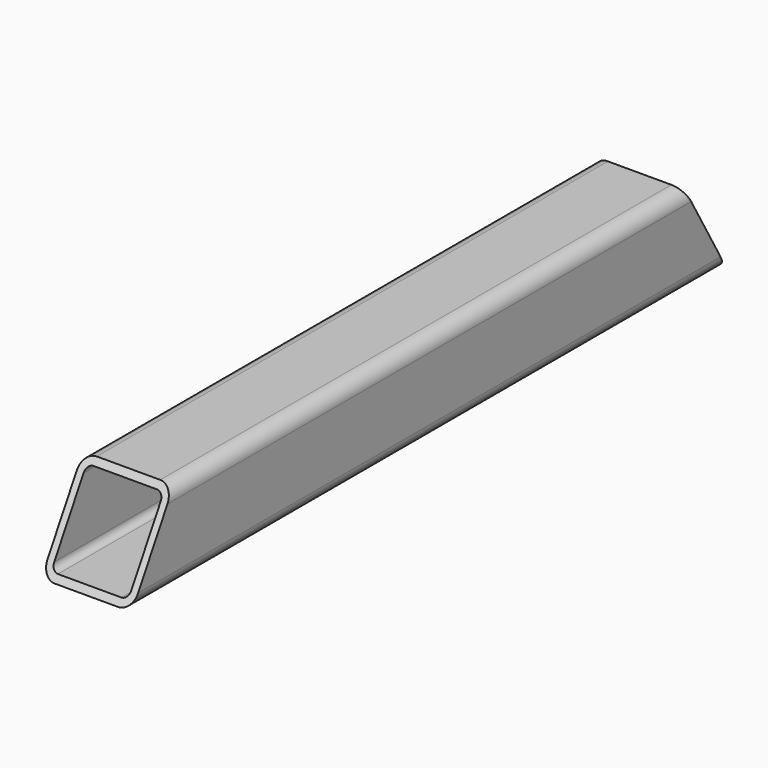
from build123d import *

# Parameters (mm, degrees)
F1_DEPTH = 1041.4
F3_DEPTH = 127.001


# Not quite as in the source:
# - a feature names something its author has since deleted; it is built from what else it names


with BuildPart() as f1:
    # F0 (on Front) → F1 (new body)
    with BuildSketch(Plane.XZ):
        with BuildLine():
            ThreePointArc((0, 19.05), (5.5796158184, 5.5796158184), (19.05, 0))
            Line((19.05, 0), (107.95, 0))
            ThreePointArc((107.95, 0), (121.4203841816, 5.5796158184), (127, 19.05))
            Line((127, 19.05), (127, 107.95))
            ThreePointArc((127, 107.95), (121.4203841816, 121.4203841816), (107.95, 127))
            Line((107.95, 127), (19.05, 127))
            ThreePointArc((19.05, 127), (5.5796158184, 121.4203841816), (0, 107.95))
            Line((0, 107.95), (0, 19.05))
        make_face()
        with BuildLine():
            ThreePointArc((19.05, 9.525), (12.3148079092, 12.3148079092), (9.525, 19.05))
            Line((9.525, 19.05), (9.525, 107.95))
            ThreePointArc((9.525, 107.95), (12.3148079092, 114.6851920908), (19.05, 117.475))
            Line((19.05, 117.475), (107.95, 117.475))
            ThreePointArc((107.95, 117.475), (114.6851920908, 114.6851920908), (117.475, 107.95))
            Line((117.475, 107.95), (117.475, 19.05))
            ThreePointArc((117.475, 19.05), (114.6851920908, 12.3148079092), (107.95, 9.525))
            Line((107.95, 9.525), (19.05, 9.525))
        make_face(mode=Mode.SUBTRACT)
    extrude(amount=F1_DEPTH)

    # F2 (on Right) → F3 (cut, through all)
    with BuildSketch(Plane.YZ):
        Polygon((-1041.4, 19.05), (-1041.4, 0), (-968.0765158129, 127), (-1041.4, 127), (-1041.4, 107.95), align=None)
        Polygon((-73.3234841871, 127), (0, 0), (0, 19.05), (0, 107.95), (0, 127), align=None)
    extrude(amount=F3_DEPTH, mode=Mode.SUBTRACT)


solid = f1.part
